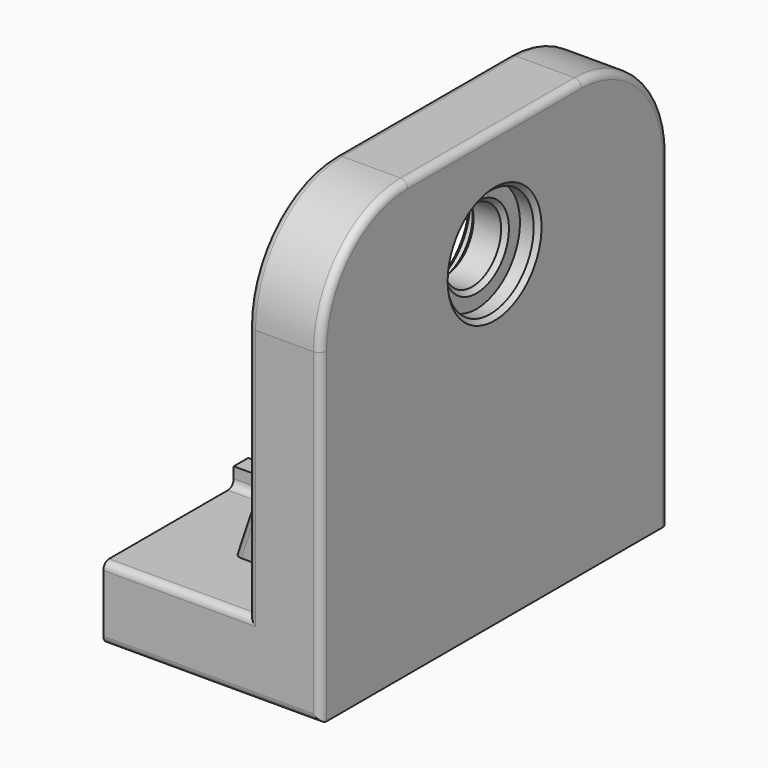
from build123d import *

# Parameters (mm, degrees)
F1_DEPTH  = 76.2
F2_R      = 12.7
F3_DEPTH  = 76.201
F5_DEPTH  = 25.401
F7_R      = 19.05
F8_DEPTH  = 6.35
F12_START = -69.85
F12_DEPTH = 12.7
F13_R     = 38.1
F14_SIZE  = 1.524
F16_DEPTH = 6.35
F17_R     = 2.54


# Not quite as in the source:
# - a pattern or mirror of a feature is missing from the dataset's text; its kind, count and spacing are read off the source's solid


with BuildPart() as f1:
    # F0 (on Front) → F1 (new body, symmetric)
    with BuildSketch(Plane.XZ):
        Polygon((0, 0), (-50.8, 0), (-50.8, -25.4), (25.4, -25.4), (25.4, 127), (0, 127), align=None)
    extrude(amount=F1_DEPTH, both=True)

    # F2 (on face) → F3 (cut, through all)
    with BuildSketch(Plane.YZ.offset(25.4)):
        with Locations((0, 88.9)):
            Circle(F2_R)
    extrude(amount=-F3_DEPTH, mode=Mode.SUBTRACT)

    # F4 (on face) → F5 (cut, through all)
    with BuildSketch(Plane.XY):
        with BuildLine():
            Line((-50.8, -12.7), (-38.1, -12.7))
            ThreePointArc((-38.1, -12.7), (-25.4, 0), (-38.1, 12.7))
            Line((-38.1, 12.7), (-50.8, 12.7))
            Line((-50.8, 12.7), (-50.8, -12.7))
        make_face()
    extrude(amount=-F5_DEPTH, mode=Mode.SUBTRACT)

    # F7 (on face) → F8 (cut)
    with BuildSketch(Plane(origin=(0, 0, 0), x_dir=(0, -1, 0), z_dir=(-1, 0, 0))):
        with Locations((0, 88.9)):
            Circle(F7_R)
    f8 = extrude(amount=-F8_DEPTH, mode=Mode.SUBTRACT)

    # F8_copies: F8 across plane
    add(f8.mirror(Plane(origin=(12.7, 0, 0), x_dir=(0, 0, 1), z_dir=(1, 0, 0))), mode=Mode.SUBTRACT)

    # F11 (on offset) → F12 (join)
    with BuildSketch(Plane.XZ.offset(120.65).offset(F12_START)):
        Polygon((0, 0), (0, 76.2), (-25.4, 0), align=None)
    f12 = extrude(amount=-F12_DEPTH)

    # F12_copies: F12 across plane
    add(f12.mirror(Plane.ZX))

    # F13
    f13_edges = [f1.edges().sort_by_distance(p)[0] for p in [
        (12.7, 76.2, 127),
        (12.7, -76.2, 127),
    ]]
    fillet(f13_edges, radius=F13_R)

    # F14
    f14_edges = [f1.edges().sort_by_distance(p)[0] for p in [
        (6.35, -12.7, 88.9),
        (0, 19.05, 88.9),
        (25.4, 19.05, 88.9),
        (19.05, -12.7, 88.9),
    ]]
    chamfer(f14_edges, length=F14_SIZE)

    # F15 (on face) → F16 (join)
    with BuildSketch(Plane.XY):
        with BuildLine():
            Line((-50.8, -19.05), (-38.1, -19.05))
            ThreePointArc((-38.1, -19.05), (-19.05, 0), (-38.1, 19.05))
            Line((-38.1, 19.05), (-50.8, 19.05))
            Line((-50.8, 19.05), (-50.8, 12.7))
            Line((-50.8, 12.7), (-38.1, 12.7))
            ThreePointArc((-38.1, 12.7), (-25.4, 0), (-38.1, -12.7))
            Line((-38.1, -12.7), (-50.8, -12.7))
            Line((-50.8, -12.7), (-50.8, -19.05))
        make_face()
    extrude(amount=F16_DEPTH)

    # F17
    f17_edges = [f1.edges().sort_by_distance(p)[0] for p in [
        (-44.45, 19.05, 0),
        (-12.7, -38.1, 38.1),
        (-12.7, -50.8, 38.1),
        (0, -76.2, 44.45),
        (25.4, -76.2, 31.75),
        (-25.4, -76.2, 0),
        (-12.7, -76.2, -25.4),
        (-25.4, 76.2, 0),
        (-12.7, 76.2, -25.4),
        (25.4, 76.2, 31.75),
        (25.4, 65.040768, 115.840768),
        (25.4, 0, 127),
        (25.4, -65.040768, 115.840768),
        (0, -65.040768, 115.840768),
        (0, 0, 127),
        (0, 65.040768, 115.840768),
        (0, 76.2, 44.45),
        (-12.7, 50.8, 38.1),
        (-12.7, 38.1, 38.1),
        (-44.45, -19.05, 0),
        (-19.05, 0, 0),
    ]]
    fillet(f17_edges, radius=F17_R)


solid = f1.part
